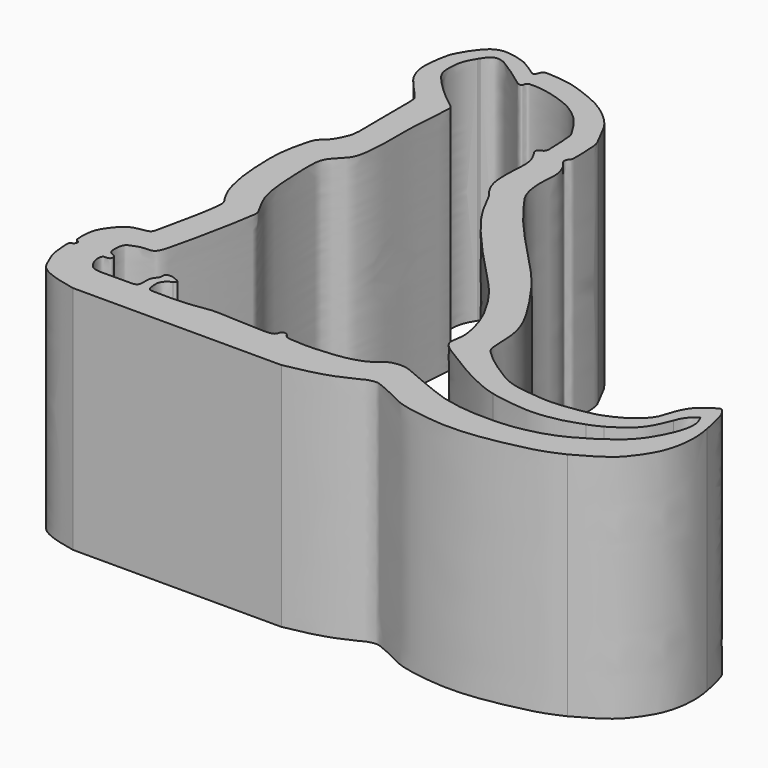
from build123d import *

# Parameters (mm, degrees)
F1_DEPTH = 10


with BuildPart() as f1:
    # F0 (on Top) → F1 (new body)
    with BuildSketch(Plane.XY):
        with BuildLine():
            add(Edge.make_bspline(
                [(-11.4531535655, 17.9316624999), (-11.3423634009, 17.8226080387), (-11.0990398713, 17.5830965577), (-10.5216537315, 17.1752428127), (-9.9832375082, 16.8116000023), (-9.3302766014, 16.5049497915), (-8.5351497911, 16.4210907342), (-7.6826916981, 16.3193589), (-6.9889404844, 16.398664447), (-6.4101964363, 16.4684482113), (-5.6925140638, 16.6154358699), (-5.2172506174, 16.8300922836), (-4.737926802, 17.0715715686), (-4.3068785624, 17.4497022766), (-4.1346039941, 17.6858196333), (-4.0643941611, 17.826827243)],
                knots=[0, 0, 0, 0, 0.042419574, 0.0931642308, 0.1423699622, 0.1931044872, 0.2473970709, 0.3037382441, 0.353898392, 0.4004323317, 0.4518808925, 0.4957535606, 0.5399514919, 0.5853730988, 0.6259275813, 0.6259275813, 0.6259275813, 0.6259275813], degree=3))
            add(Edge.make_bspline(
                [(-11.4531535655, 17.9316624999), (-11.5353278284, 18.0013325693), (-11.599494506, 18.1546413097), (-11.6392459174, 18.4329153399), (-11.6321864133, 19.5729774369), (-12.121309762, 20.7408570607), (-13.2308142182, 22.3617998661), (-13.8442255961, 23.2013966392), (-16.3773954957, 25.7550440824), (-17.205806736, 26.9338284954), (-17.893694871, 27.7744469667), (-17.9002010475, 29.021400573), (-17.8184822247, 29.5057983061), (-17.9897855014, 30.0497916449), (-18.1881615527, 30.275766195), (-18.2946934326, 30.4049965252), (-18.2620452332, 30.5813836452), (-18.1277397895, 30.6574477694), (-18.1285761686, 31.0906791932), (-18.1624494507, 31.9344986736), (-18.2120670314, 32.1457449013), (-18.2822644711, 32.2766117752)],
                knots=[0.1821779851, 0.1821779851, 0.1821779851, 0.1821779851, 0.1987968455, 0.2156710174, 0.2494905898, 0.2877760322, 0.3323884407, 0.3678427424, 0.4293232275, 0.4698632522, 0.5029651526, 0.5385501207, 0.5620196375, 0.58602784, 0.6039449868, 0.6168302331, 0.629630365, 0.6412448386, 0.6621791519, 0.6923850095, 0.7125211911, 0.7125211911, 0.7125211911, 0.7125211911], degree=3))
            add(Edge.make_bspline(
                [(-18.2822644711, 32.2766117752), (-18.3764124539, 32.4691395294), (-18.5746716934, 32.8745694176), (-18.9547100724, 33.5767458928), (-19.8713796985, 34.3090133343), (-20.6712786085, 34.6655738311), (-21.5630569798, 34.9977244911), (-22.289607185, 35.0857544204), (-22.739681166, 35.1104890737), (-22.8902895116, 35.0922607106), (-22.9567494288, 34.9547105739), (-22.9959628259, 34.85761112), (-23.0162381196, 34.789313499), (-23.0410310579, 34.7767824349), (-23.0424862006, 34.7761286919)],
                knots=[0, 0, 0, 0, 0.0875488863, 0.1843626926, 0.3004828811, 0.4033844393, 0.5086232519, 0.6027505646, 0.6738982423, 0.7129539346, 0.7530518454, 0.7894959828, 0.8210273533, 0.8229308962, 0.8229308962, 0.8229308962, 0.8229308962], degree=3))
            add(Edge.make_bspline(
                [(-23.0424862006, 34.7761286919), (-23.0449273652, 34.7750319649), (-23.0474912695, 34.7741032154), (-23.0501528602, 34.7733159161)],
                knots=[0.8229308962, 0.8229308962, 0.8229308962, 0.8229308962, 0.8261243023, 0.8261243023, 0.8261243023, 0.8261243023], degree=3))
            add(Edge.make_bspline(
                [(-23.0501528602, 34.7733159161), (-23.0545410802, 34.7718037439), (-23.0658169935, 34.7685198591), (-23.0800204513, 34.7682348796), (-23.0884888755, 34.7688855933)],
                knots=[0.0021581351, 0.0021581351, 0.0021581351, 0.0021581351, 0.005798454, 0.0111263901, 0.0111263901, 0.0111263901, 0.0111263901], degree=3))
            add(Edge.make_bspline(
                [(-23.0884888755, 34.7688855933), (-23.1003779199, 34.7686586533), (-23.1328950749, 34.7691224435), (-23.1675617858, 34.7535809385), (-23.1907266171, 34.8047911582), (-23.2061327949, 34.8275179634)],
                knots=[0.8400573422, 0.8400573422, 0.8400573422, 0.8400573422, 0.8525582929, 0.8747680855, 0.9015857102, 0.9015857102, 0.9015857102, 0.9015857102], degree=3))
            add(Edge.make_bspline(
                [(-23.2061327949, 34.8275179634), (-23.2333559253, 34.8463304823), (-23.2647020116, 34.8687780005), (-23.2981565972, 34.8923575129)],
                knots=[0.0280714161, 0.0280714161, 0.0280714161, 0.0280714161, 0.0354838753, 0.0354838753, 0.0354838753, 0.0354838753], degree=3))
            add(Edge.make_bspline(
                [(-23.2981565972, 34.8923575129), (-23.2988767288, 34.892762275), (-23.3248742022, 34.9074866854), (-23.3553511069, 34.9290724478), (-23.3874430501, 34.9538305609)],
                knots=[0.9407451714, 0.9407451714, 0.9407451714, 0.9407451714, 0.9414461456, 0.9659304091, 0.9659304091, 0.9659304091, 0.9659304091], degree=3))
            add(Edge.make_bspline(
                [(-23.3874430501, 34.9538305609), (-23.3931059977, 34.9575991511), (-23.5183257902, 35.0402229402), (-23.6443291251, 35.1054632176), (-23.7584039569, 35.1838432252)],
                knots=[0.0418291952, 0.0418291952, 0.0418291952, 0.0418291952, 0.0430086944, 0.0678657162, 0.0678657162, 0.0678657162, 0.0678657162], degree=3))
            add(Edge.make_bspline(
                [(-26.1538624763, 34.1210328043), (-26.1307370492, 34.1751880638), (-26.0822982029, 34.2886224609), (-25.9658399245, 34.4784520857), (-25.8367286637, 34.7222051807), (-25.6728345837, 34.9333072266), (-25.4439024159, 35.211302267), (-25.2265629641, 35.3669839468), (-24.9870615601, 35.4455267206), (-24.8071553611, 35.4561515908), (-24.6253811619, 35.4452719932), (-24.4282528156, 35.4124563816), (-24.2023609898, 35.3568568595), (-23.9138114794, 35.2698461332), (-23.8380879164, 35.2283194661), (-23.7584039569, 35.1838432252)],
                knots=[0, 0, 0, 0, 0.0671677149, 0.1421214746, 0.2249641321, 0.3079903593, 0.4027612882, 0.4853187471, 0.5636684732, 0.6308045814, 0.6978681882, 0.7682230286, 0.8464364216, 0.9304502691, 1, 1, 1, 1], degree=3))
            add(Edge.make_bspline(
                [(-25.1203924417, 30.8839287609), (-25.1562608207, 30.9362134154), (-25.2475018018, 31.0692136602), (-25.5941633097, 31.4371340123), (-26.0988037641, 31.9831774136), (-26.3235628346, 32.5710825271), (-26.3308719409, 33.0580330838), (-26.267644153, 33.6751860491), (-26.1899151296, 33.9797626196), (-26.1538624763, 34.1210328043)],
                knots=[0, 0, 0, 0, 0.0919674503, 0.2339442329, 0.409585968, 0.566381973, 0.7063931007, 0.8638178216, 1, 1, 1, 1], degree=3))
            add(Edge.make_bspline(
                [(-25.1203924417, 30.8839287609), (-25.0886757261, 30.8488100619), (-25.0858553072, 30.7298281237), (-25.0605183202, 30.5414498556), (-25.0811840994, 29.4385381855), (-25.025121507, 27.8856571604), (-25.0878508685, 27.3842583921), (-25.2783239246, 27.0108607833), (-25.3896626652, 26.7964370834), (-25.5940210314, 26.5788191515), (-25.8230618275, 26.4054110505), (-25.9629958258, 25.978131493), (-26.1101708802, 25.2629515982), (-26.1930934834, 24.6887465002), (-26.1587460044, 23.5953713197), (-26.0923778546, 22.7066225224), (-25.8549842087, 21.6428561237), (-25.4792186965, 21.0084943162), (-25.2488940087, 20.7558964092), (-25.6031770536, 19.1423379832), (-25.8752014488, 17.9034210742)],
                knots=[0.445949678, 0.445949678, 0.445949678, 0.445949678, 0.4606016519, 0.4767201663, 0.5169581501, 0.5660347046, 0.5932453766, 0.6172063162, 0.6362765888, 0.6569197902, 0.677099802, 0.7025270895, 0.7352531162, 0.7651894637, 0.8048239261, 0.8421337262, 0.8826114218, 0.9145317439, 0.9341388234, 1, 1, 1, 1], degree=3))
            add(Edge.make_bspline(
                [(-25.8752014488, 17.9034210742), (-25.890226418, 17.8385940614), (-25.9181016975, 17.7183228602), (-26.0280658323, 17.6086152498), (-26.3580697207, 17.5628266856), (-26.8372170059, 17.4724464527), (-27.3412522543, 16.8823959482), (-27.5876734804, 16.3942447708), (-27.5859384154, 15.7548281184), (-27.559666492, 15.6041924875), (-27.4454298624, 15.5597037984), (-27.4091925648, 15.5164474494), (-27.40446379, 15.4213679956), (-27.4685753547, 15.3262476594), (-27.5338586836, 15.3167507729), (-27.6002461641, 15.2885968197), (-27.6332812217, 15.1859599479), (-27.5983987717, 14.8301530597), (-27.5615282937, 14.3707910049), (-27.4634080296, 14.0958808888), (-27.3264889208, 13.8151837564), (-27.1982899269, 13.4630176243), (-26.9092353443, 13.1931500637), (-26.4150422105, 13.0016663658), (-26.1029425206, 12.9146269902), (-25.6877393944, 12.8221827022), (-25.4437103868, 12.765155333)],
                knots=[0, 0, 0, 0, 0.0344863373, 0.0639855733, 0.1086241936, 0.1641824578, 0.2327490814, 0.2937225355, 0.3559622593, 0.3853098427, 0.4111499512, 0.4294614236, 0.4532568552, 0.4793434925, 0.499421999, 0.5194489997, 0.5434180278, 0.5910075895, 0.64611278, 0.688915408, 0.7331184434, 0.7813380609, 0.8313225626, 0.8883414874, 0.9343006116, 1, 1, 1, 1], degree=3))
            Line((-25.4437103868, 12.765155333), (-16.4025947478, 12.765155333))
            add(Edge.make_bspline(
                [(-16.4025947478, 12.765155333), (-16.1325477154, 12.8121301717), (-15.6410122013, 12.9046834632), (-14.9844065574, 13.0825012477), (-14.3633058233, 13.2783819833), (-13.5688307679, 13.6611160533), (-13.4493540543, 13.7432549192), (-13.1147097273, 13.8045320217), (-12.93922772, 13.7837422569), (-12.1480315577, 13.437274029), (-11.5088259607, 13.0448039918), (-10.2445374068, 12.8357133347), (-9.1498502359, 12.7336593824), (-7.965074114, 12.8220975242), (-6.8232223523, 13.03483049), (-5.6038998247, 13.3021566911), (-4.9807119282, 13.5887327234), (-4.7370914961, 13.6951681509)],
                knots=[0, 0, 0, 0, 0.0553291926, 0.1059431332, 0.158535845, 0.2156720776, 0.2406225556, 0.27495853, 0.3021246856, 0.3581217371, 0.4143329098, 0.4838231748, 0.550330998, 0.6177137492, 0.6856038145, 0.7557468163, 0.8158364686, 0.8158364686, 0.8158364686, 0.8158364686], degree=3))
            add(Edge.make_bspline(
                [(-4.7370914961, 13.6951681509), (-4.6336168572, 13.7497695407), (-4.4022190396, 13.8718733002), (-3.915698601, 14.1583931236), (-3.3189609958, 14.5578766942), (-2.8415437902, 15.1210480371), (-2.393185713, 15.8326132355), (-2.1726225731, 16.5980120919), (-2.106400575, 17.3823937336), (-2.1753231615, 17.9085416842), (-2.2190036252, 18.1177239865)],
                knots=[0, 0, 0, 0, 0.0743850462, 0.1663454691, 0.2702248812, 0.3756822507, 0.4875855348, 0.5966665154, 0.7059543766, 0.810481295, 0.810481295, 0.810481295, 0.810481295], degree=3))
            add(Edge.make_bspline(
                [(-2.2190036252, 18.1177239865), (-2.2518107461, 18.2748347059), (-2.3191938065, 18.5027389298), (-2.4290399311, 18.6979265504), (-2.5020790265, 18.7794991688), (-2.5303655878, 18.8093540446)],
                knots=[0.810481295, 0.810481295, 0.810481295, 0.810481295, 0.8889884113, 0.9480975652, 0.9842665566, 0.9842665566, 0.9842665566, 0.9842665566], degree=3))
            add(Edge.make_bspline(
                [(-2.5303655878, 18.8093540446), (-2.5426701888, 18.8223408596), (-2.5550807251, 18.8351173916), (-2.5674912613, 18.8478939235)],
                knots=[0.9842665566, 0.9842665566, 0.9842665566, 0.9842665566, 1, 1, 1, 1], degree=3))
            add(Edge.make_bspline(
                [(-4.0643941611, 17.826827243), (-3.9865836201, 17.9830999177), (-3.86768057, 18.3397290309), (-3.6416754276, 18.6704218123), (-3.3503084939, 18.8584432296), (-3.0550237105, 18.9017134543), (-2.7920699812, 18.9152360919), (-2.6246045598, 18.893669034), (-2.5674912613, 18.8478939235)],
                knots=[0.6259275813, 0.6259275813, 0.6259275813, 0.6259275813, 0.6708723716, 0.7091205339, 0.7439142078, 0.7767324746, 0.8080795091, 0.8368777612, 0.8368777612, 0.8368777612, 0.8368777612], degree=3))
        make_face()
        with BuildLine():
            add(Edge.make_bspline(
                [(-18.6367090791, 26.806615293), (-18.8379953623, 27.065709235), (-19.2790347915, 27.6334113281), (-19.1385849927, 29.1576934988), (-19.142782507, 29.5768376419), (-19.2364724588, 29.9460879236), (-19.432292799, 30.245707849), (-19.5036923614, 30.3711508025), (-19.452039249, 30.531044358), (-19.1832908953, 30.5779669697), (-19.2042061287, 31.0575192756), (-19.2501349062, 31.946730439), (-19.3048676283, 32.1518750406), (-19.8206112027, 32.9401597753), (-20.1781911638, 33.2766280139), (-20.6657936013, 33.6375280434), (-21.1987273574, 33.8502544994), (-21.8156732253, 34.0369903903), (-22.3532940037, 34.1202740074), (-22.6789525507, 34.1114092951), (-22.781036981, 34.0935154005), (-22.8442123538, 34.0064923878), (-22.836017646, 33.8992917505), (-22.9169687736, 33.8654371785), (-23.0415440189, 33.8778928228), (-23.145046001, 33.9920059469), (-24.3172951647, 34.8056332509), (-24.4709784088, 34.846264388), (-24.6665006085, 34.9235282636), (-24.8730036275, 34.8890028633), (-25.0225147118, 34.7975179285), (-25.1513236902, 34.5965507599), (-25.1965038478, 34.5278270543)],
                knots=[0, 0, 0, 0, 0.0530449929, 0.1162271616, 0.1503362798, 0.1818999441, 0.2130503431, 0.2322815435, 0.2514640261, 0.275217638, 0.3099088569, 0.3591170068, 0.3848334384, 0.4340298475, 0.4724784579, 0.512097197, 0.5519606878, 0.5941304956, 0.6332780537, 0.6623280229, 0.6782450968, 0.6944721334, 0.7106995421, 0.7248499144, 0.7417640264, 0.7633659926, 0.8252786224, 0.8481238707, 0.8706340609, 0.8940154935, 0.9161281592, 0.9453600325, 0.9453600325, 0.9453600325, 0.9453600325], degree=3))
            add(Edge.make_bspline(
                [(-18.6367090791, 26.806615293), (-18.4004431072, 26.3177446993), (-17.8214250743, 25.1196658343), (-14.9958562057, 22.1558553104), (-14.2006384351, 21.3463203299), (-13.4069219143, 20.1028170279), (-13.057819762, 19.1966099457), (-12.8449499507, 18.2061038352), (-13.1501738463, 17.4728388827), (-12.0668415899, 16.9062569537), (-11.2465699819, 16.3394149694), (-10.3042035411, 15.8914402394), (-9.8099199153, 15.6800453052), (-9.4957305118, 15.6079921871)],
                knots=[0, 0, 0, 0, 0.070520737, 0.1729047088, 0.2297494243, 0.2895443737, 0.3410861891, 0.3916345783, 0.432452015, 0.4846611235, 0.5378002653, 0.5889842833, 0.636687273, 0.636687273, 0.636687273, 0.636687273], degree=3))
            add(Edge.make_bspline(
                [(-9.4957305118, 15.6079921871), (-9.1133312834, 15.5202964964), (-8.2008881683, 15.4402897436), (-7.3081707518, 15.4279642007), (-6.2775050816, 15.7326586203), (-5.5702812914, 15.970748713), (-5.1639379173, 16.0504758378), (-5.0442288589, 16.0616629529)],
                knots=[0.636687273, 0.636687273, 0.636687273, 0.636687273, 0.6947464763, 0.7437941737, 0.7961098113, 0.8448976449, 0.8661305735, 0.8661305735, 0.8661305735, 0.8661305735], degree=3))
            add(Edge.make_bspline(
                [(-5.0442288589, 16.0616629529), (-4.9399228548, 16.1184542498), (-4.6922932366, 16.2700279948), (-4.3072979632, 16.5467521861), (-3.9111782293, 16.9402090766), (-3.6467479793, 17.4860351741), (-3.5418440062, 17.7515041171), (-3.4855501726, 17.880808562)],
                knots=[0.1116059668, 0.1116059668, 0.1116059668, 0.1116059668, 0.174466562, 0.2640043057, 0.3569942582, 0.452966765, 0.5340334981, 0.5340334981, 0.5340334981, 0.5340334981], degree=3))
            add(Edge.make_bspline(
                [(-3.4855501726, 17.880808562), (-3.4648551188, 17.9392815903), (-3.4254729985, 18.0505541605), (-3.3592609609, 18.1784369474), (-3.2239072693, 18.3745123065), (-3.075018802, 18.5162428051), (-2.960889175, 18.580902775), (-2.9049660079, 18.6125859618)],
                knots=[0, 0, 0, 0, 0.1933263651, 0.3678947746, 0.5897403457, 0.798974028, 1, 1, 1, 1], degree=3))
            add(Edge.make_bspline(
                [(-2.7946273377, 18.3692199386), (-2.7964008531, 18.3746177266), (-2.8185376651, 18.4405657555), (-2.8607845108, 18.5367806837), (-2.8920297064, 18.5903902465), (-2.9049660079, 18.6125859618)],
                knots=[0.7742104558, 0.7742104558, 0.7742104558, 0.7742104558, 0.7853442377, 0.9111270835, 1, 1, 1, 1], degree=3))
            add(Edge.make_bspline(
                [(-2.7946273377, 18.3692199386), (-2.7819962135, 18.3572528177), (-2.7467831192, 18.3156041133), (-2.6954959966, 18.2431388933), (-2.7118146433, 18.0844860008), (-2.7163067479, 18.0028985872), (-2.7269718703, 17.9558321834)],
                knots=[0.7904142153, 0.7904142153, 0.7904142153, 0.7904142153, 0.8091254065, 0.8492766078, 0.8974005007, 0.94294828, 0.94294828, 0.94294828, 0.94294828], degree=3))
            add(Edge.make_bspline(
                [(-2.7589141579, 17.8106968769), (-2.7480705925, 17.8589856053), (-2.7375212314, 17.9074088943), (-2.7269718703, 17.9558321834)],
                knots=[0.9678475586, 0.9678475586, 0.9678475586, 0.9678475586, 1, 1, 1, 1], degree=3))
            add(Edge.make_bspline(
                [(-2.8583404767, 17.4271704529), (-2.8514740504, 17.4479914895), (-2.8244370396, 17.5313499213), (-2.7886322661, 17.653954814), (-2.7657065006, 17.7682841548), (-2.7589141579, 17.8106968769)],
                knots=[0.0876086045, 0.0876086045, 0.0876086045, 0.0876086045, 0.1340096964, 0.2726867204, 0.3537768689, 0.3537768689, 0.3537768689, 0.3537768689], degree=3))
            add(Edge.make_bspline(
                [(-2.8978604823, 17.3097904772), (-2.8837879349, 17.3485058616), (-2.8706743906, 17.3876598669), (-2.8583404767, 17.4271704529)],
                knots=[0.8542372602, 0.8542372602, 0.8542372602, 0.8542372602, 0.8815008623, 0.8815008623, 0.8815008623, 0.8815008623], degree=3))
            add(Edge.make_bspline(
                [(-4.1314834672, 15.5965547193), (-4.0315274216, 15.6733263507), (-3.7778639874, 15.8777413762), (-3.4320979017, 16.2764907518), (-3.160297974, 16.7462504522), (-2.970488838, 17.1099805481), (-2.8978604823, 17.3097904772)],
                knots=[0.3513635715, 0.3513635715, 0.3513635715, 0.3513635715, 0.4468641765, 0.5821895305, 0.71352993, 0.8542372602, 0.8542372602, 0.8542372602, 0.8542372602], degree=3))
            add(Edge.make_bspline(
                [(-5.1270611584, 14.938313514), (-5.0515530743, 14.9774552199), (-4.8843674391, 15.0641205227), (-4.5469469405, 15.2867318902), (-4.3174529957, 15.4558821713), (-4.1670458139, 15.5692409199), (-4.1314834672, 15.5965547193)],
                knots=[0, 0, 0, 0, 0.092613947, 0.2050604481, 0.3173863808, 0.3513635715, 0.3513635715, 0.3513635715, 0.3513635715], degree=3))
            add(Edge.make_bspline(
                [(-5.1270611584, 14.938313514), (-5.2771142269, 14.8341591333), (-5.6563184579, 14.6364611177), (-6.2827280989, 14.3709318177), (-7.113865798, 14.1755257038), (-7.8061594564, 14.0723005413), (-8.7575945258, 14.062762844), (-9.4755779778, 14.0903441294), (-10.5171680112, 14.2640694268), (-11.0849865282, 14.495208914), (-11.6394734923, 14.7117769501), (-12.3199132485, 14.9929642703), (-12.7929010289, 15.2160549407), (-13.1693051019, 15.3094794414), (-13.6631097568, 15.2406991201), (-13.8878987376, 15.0699376691), (-14.1270175817, 14.8596805039), (-14.4365379063, 14.6998032363), (-14.946365692, 14.5441603648), (-15.4653725357, 14.4701314227), (-16.0228531057, 14.4259051639), (-16.599280406, 14.3831817298), (-17.1563207893, 14.4291134823), (-17.5765573618, 14.4432909445), (-17.6426388891, 14.6781332324), (-17.9252680634, 14.7019285451), (-17.9369295949, 14.4385445784), (-18.1966937306, 14.3022551156), (-19.2514603507, 14.3796871572), (-20.1516024839, 14.4031902832), (-20.7000563565, 14.4503697732), (-21.2012371276, 14.346136563), (-21.6956016992, 14.2977665359), (-22.2745615473, 14.2463720239), (-22.9643071169, 14.2929417537), (-23.4041762898, 14.2443440285), (-23.4357489045, 14.6405144544), (-23.4448194595, 14.9162666216), (-23.2529802358, 15.1376544408), (-23.1260398226, 15.2011345711), (-23.0670906603, 15.2306137607)],
                knots=[0.2264805435, 0.2264805435, 0.2264805435, 0.2264805435, 0.2486079389, 0.2725642119, 0.2988704638, 0.3232808251, 0.3508193168, 0.3758397165, 0.4050386993, 0.427596275, 0.4496366082, 0.4744321143, 0.4951166283, 0.5129757033, 0.5327762454, 0.5479843164, 0.5638359997, 0.5807872712, 0.6016612368, 0.6226275802, 0.6440520809, 0.6659820881, 0.6879120602, 0.7054182805, 0.7182618618, 0.7311197199, 0.7440164781, 0.7580595368, 0.787518082, 0.8155871711, 0.8365634894, 0.8567932415, 0.8769411061, 0.899021601, 0.9233900622, 0.9405536451, 0.956742594, 0.9720531433, 0.9869513902, 1, 1, 1, 1], degree=3))
            add(Edge.make_bspline(
                [(-25.2310526286, 34.4719983222), (-25.3038391294, 34.3540012216), (-25.4531529498, 34.1042935473), (-25.5721470358, 33.7092541942), (-25.587188472, 33.1298241951), (-25.4997983265, 32.7713027421), (-25.0413920552, 32.246510563), (-24.405800543, 31.6505354237), (-23.897365776, 31.2578208694), (-23.7384603201, 31.1382864161), (-23.6760367082, 30.9234858301), (-23.8646136174, 29.371515056), (-23.8160584786, 27.8408048298), (-23.8551271681, 27.1541425133), (-23.9417054048, 26.339591915), (-24.1841815052, 26.0016383593), (-24.5166982086, 25.6736562258), (-24.7714149026, 25.3473157244), (-24.8024256704, 24.6413497116), (-24.7578308739, 23.6496523325), (-24.6946622518, 22.7425708957), (-24.5195394508, 21.8598876019), (-24.0198688435, 21.0761443867), (-23.9591596225, 20.7748494681), (-24.7186554159, 17.060654472), (-24.8645659656, 16.776896027), (-25.0058611967, 16.5379639168), (-25.4743029949, 16.5886627468), (-25.828810169, 16.422282137), (-26.117255434, 16.3440434258), (-26.1701546323, 15.6477142433), (-25.960334184, 15.551537143), (-25.7824829921, 15.4608173801), (-25.7700435102, 15.2730663669), (-25.9120797072, 15.1993096117), (-26.120103391, 15.2497938765), (-26.1587468696, 14.9656310604), (-26.1025293294, 14.7432897715), (-25.9857633015, 14.511549356), (-25.8184734838, 14.331032355), (-25.6147179493, 14.2801439987), (-25.3514809746, 14.2616198502), (-24.4496681404, 14.2701286396), (-24.0407142438, 14.2676187035), (-23.8240741539, 14.3523693205), (-23.8551603339, 14.7361797958), (-23.8173415435, 15.0196417279), (-23.5949082397, 15.2256291566), (-23.6362962994, 15.4703033213), (-23.5144593574, 15.5291150345), (-23.3262235385, 15.5282810576), (-23.1721817841, 15.4584836678), (-22.9132569839, 15.3623304285), (-23.0186889838, 15.2720566209), (-23.0670906603, 15.2306137607)],
                knots=[0.0027278011, 0.0027278011, 0.0027278011, 0.0027278011, 0.0200249886, 0.0393548678, 0.0612294478, 0.0786838853, 0.1025489241, 0.1307470779, 0.1538969322, 0.1658959497, 0.1780571677, 0.2142283318, 0.2513672974, 0.2758186495, 0.3014641695, 0.3202193243, 0.3398196416, 0.3581136586, 0.3821190631, 0.4115331974, 0.439462177, 0.467632387, 0.4942257926, 0.5124318159, 0.5686189168, 0.5863858262, 0.5995567566, 0.6189060586, 0.6372612295, 0.6522652849, 0.6748270314, 0.6879979824, 0.7005384814, 0.7118123465, 0.7226500232, 0.7346799252, 0.7485649543, 0.7629617211, 0.7777715626, 0.7920285271, 0.8046940387, 0.8198234075, 0.84771286, 0.866790111, 0.878951312, 0.8961848444, 0.9120081261, 0.9274768414, 0.9408689641, 0.9504318938, 0.9627680851, 0.9755932763, 0.9887953719, 1, 1, 1, 1], degree=3))
            add(Edge.make_bspline(
                [(-25.1965038478, 34.5278270543), (-25.2109680444, 34.5058255111), (-25.2225466217, 34.4885071169), (-25.2310526286, 34.4719983222)],
                knots=[0.9453600325, 0.9453600325, 0.9453600325, 0.9453600325, 0.9547184674, 0.9547184674, 0.9547184674, 0.9547184674], degree=3))
        make_face(mode=Mode.SUBTRACT)
        with BuildLine():
            add(Edge.make_bspline(
                [(-4.0643941611, 17.826827243), (-4.0329021527, 17.9274360865), (-3.9633756818, 18.1495552272), (-3.8023122301, 18.6095361712), (-3.555300918, 19.0266262674), (-3.1821771361, 19.322271683), (-2.9551182407, 19.4661996221), (-2.846354153, 19.5351429284)],
                knots=[0, 0, 0, 0, 0.1756674888, 0.38782984, 0.6003192445, 0.8085478544, 1, 1, 1, 1], degree=3))
            add(Edge.make_bspline(
                [(-4.0643941611, 17.826827243), (-3.9865836201, 17.9830999177), (-3.86768057, 18.3397290309), (-3.6416754276, 18.6704218123), (-3.3503084939, 18.8584432296), (-3.0550237105, 18.9017134543), (-2.7920699812, 18.9152360919), (-2.6246045598, 18.893669034), (-2.5674912613, 18.8478939235)],
                knots=[0.6259275813, 0.6259275813, 0.6259275813, 0.6259275813, 0.6708723716, 0.7091205339, 0.7439142078, 0.7767324746, 0.8080795091, 0.8368777612, 0.8368777612, 0.8368777612, 0.8368777612], degree=3))
            add(Edge.make_bspline(
                [(-2.5674912613, 18.8478939235), (-2.5538474608, 18.8369587037), (-2.5415202907, 18.824000489), (-2.5303655878, 18.8093540446)],
                knots=[0.8368777612, 0.8368777612, 0.8368777612, 0.8368777612, 0.843757378, 0.843757378, 0.843757378, 0.843757378], degree=3))
            add(Edge.make_bspline(
                [(-2.2190036252, 18.1177239865), (-2.2518107461, 18.2748347059), (-2.3191938065, 18.5027389298), (-2.4290399311, 18.6979265504), (-2.5020790265, 18.7794991688), (-2.5303655878, 18.8093540446)],
                knots=[0.810481295, 0.810481295, 0.810481295, 0.810481295, 0.8889884113, 0.9480975652, 0.9842665566, 0.9842665566, 0.9842665566, 0.9842665566], degree=3))
            add(Edge.make_bspline(
                [(-2.2190036252, 18.1177239865), (-2.2295599779, 18.1909128286), (-2.2525944027, 18.350614094), (-2.3311223768, 18.6665866168), (-2.411011017, 18.9856929483), (-2.5034334632, 19.2962170954), (-2.6620392862, 19.4790050752), (-2.699362075, 19.5283454236), (-2.7892871387, 19.5677127173), (-2.8284091094, 19.5453846817), (-2.846354153, 19.5351429284)],
                knots=[0, 0, 0, 0, 0.1385698593, 0.3023655142, 0.469346878, 0.6353465435, 0.772083198, 0.8437606813, 0.9283338407, 1, 1, 1, 1], degree=3))
        make_face()
        with BuildLine():
            add(Edge.make_bspline(
                [(-9.4957305118, 15.6079921871), (-9.1133312834, 15.5202964964), (-8.2008881683, 15.4402897436), (-7.3081707518, 15.4279642007), (-6.2775050816, 15.7326586203), (-5.5702812914, 15.970748713), (-5.1639379173, 16.0504758378), (-5.0442288589, 16.0616629529)],
                knots=[0.636687273, 0.636687273, 0.636687273, 0.636687273, 0.6947464763, 0.7437941737, 0.7961098113, 0.8448976449, 0.8661305735, 0.8661305735, 0.8661305735, 0.8661305735], degree=3))
            add(Edge.make_bspline(
                [(-9.4957305118, 15.6079921871), (-9.2948678262, 15.5463206649), (-8.7000059095, 15.4649529633), (-7.7290203732, 15.3419949223), (-6.8886297907, 15.4400960431), (-6.2129135882, 15.5896585333), (-5.8190504445, 15.747745542), (-5.6177424267, 15.8075205982)],
                knots=[0, 0, 0, 0, 0.0254322528, 0.0542807701, 0.0806860867, 0.1044391847, 0.1272162238, 0.1272162238, 0.1272162238, 0.1272162238], degree=3))
            add(Edge.make_bspline(
                [(-5.6177424267, 15.8075205982), (-5.466753069, 15.8664520418), (-5.2723213776, 15.9423391137), (-5.0856063663, 16.039134218), (-5.0442288589, 16.0616629529)],
                knots=[0, 0, 0, 0, 0.0866695811, 0.1116059668, 0.1116059668, 0.1116059668, 0.1116059668], degree=3))
        make_face()
        with BuildLine():
            add(Edge.make_bspline(
                [(-2.7946273377, 18.3692199386), (-2.7819962135, 18.3572528177), (-2.7467831192, 18.3156041133), (-2.6954959966, 18.2431388933), (-2.7118146433, 18.0844860008), (-2.7163067479, 18.0028985872), (-2.7269718703, 17.9558321834)],
                knots=[0.7904142153, 0.7904142153, 0.7904142153, 0.7904142153, 0.8091254065, 0.8492766078, 0.8974005007, 0.94294828, 0.94294828, 0.94294828, 0.94294828], degree=3))
            add(Edge.make_bspline(
                [(-2.7498320277, 17.8763530796), (-2.7482850512, 17.8897743927), (-2.7401795828, 17.9706760352), (-2.7408634662, 18.0956768484), (-2.745224744, 18.1928070831), (-2.7747005451, 18.308571691), (-2.7946273377, 18.3692199386)],
                knots=[0.3956408743, 0.3956408743, 0.3956408743, 0.3956408743, 0.4214109088, 0.5516550538, 0.64911396, 0.7742104558, 0.7742104558, 0.7742104558, 0.7742104558], degree=3))
            add(Edge.make_bspline(
                [(-2.7269718703, 17.9558321834), (-2.7325770316, 17.931095966), (-2.7405247135, 17.9043172658), (-2.7498320277, 17.8763530796)],
                knots=[0.94294828, 0.94294828, 0.94294828, 0.94294828, 0.9668863692, 0.9668863692, 0.9668863692, 0.9668863692], degree=3))
        make_face()
        with BuildLine():
            add(Edge.make_bspline(
                [(-23.0884888755, 34.7688855933), (-23.1003779199, 34.7686586533), (-23.1328950749, 34.7691224435), (-23.1675617858, 34.7535809385), (-23.1907266171, 34.8047911582), (-23.2061327949, 34.8275179634)],
                knots=[0.8400573422, 0.8400573422, 0.8400573422, 0.8400573422, 0.8525582929, 0.8747680855, 0.9015857102, 0.9015857102, 0.9015857102, 0.9015857102], degree=3))
            add(Edge.make_bspline(
                [(-23.0884888755, 34.7688855933), (-23.0908912433, 34.7690701912), (-23.1071818944, 34.7707677433), (-23.1325886424, 34.7781756239), (-23.1815038199, 34.8104981332), (-23.2061327949, 34.8275179634)],
                knots=[0.0111263901, 0.0111263901, 0.0111263901, 0.0111263901, 0.0126378475, 0.0213653073, 0.0280714161, 0.0280714161, 0.0280714161, 0.0280714161], degree=3))
        make_face()
        with BuildLine():
            add(Edge.make_bspline(
                [(-2.7589141579, 17.8106968769), (-2.7480705925, 17.8589856053), (-2.7375212314, 17.9074088943), (-2.7269718703, 17.9558321834)],
                knots=[0.9678475586, 0.9678475586, 0.9678475586, 0.9678475586, 1, 1, 1, 1], degree=3))
            add(Edge.make_bspline(
                [(-2.7269718703, 17.9558321834), (-2.7325770316, 17.931095966), (-2.7405247135, 17.9043172658), (-2.7498320277, 17.8763530796)],
                knots=[0.94294828, 0.94294828, 0.94294828, 0.94294828, 0.9668863692, 0.9668863692, 0.9668863692, 0.9668863692], degree=3))
            add(Edge.make_bspline(
                [(-2.7589141579, 17.8106968769), (-2.7554075091, 17.8325930808), (-2.7523451261, 17.854549852), (-2.7498320277, 17.8763530796)],
                knots=[0.3537768689, 0.3537768689, 0.3537768689, 0.3537768689, 0.3956408743, 0.3956408743, 0.3956408743, 0.3956408743], degree=3))
        make_face()
        with BuildLine():
            add(Edge.make_bspline(
                [(-23.2981565972, 34.8923575129), (-23.2988767288, 34.892762275), (-23.3248742022, 34.9074866854), (-23.3553511069, 34.9290724478), (-23.3874430501, 34.9538305609)],
                knots=[0.9407451714, 0.9407451714, 0.9407451714, 0.9407451714, 0.9414461456, 0.9659304091, 0.9659304091, 0.9659304091, 0.9659304091], degree=3))
            add(Edge.make_bspline(
                [(-23.2981565972, 34.8923575129), (-23.3267948721, 34.9125423858), (-23.3569782443, 34.9335567781), (-23.3874430501, 34.9538305609)],
                knots=[0.0354838753, 0.0354838753, 0.0354838753, 0.0354838753, 0.0418291952, 0.0418291952, 0.0418291952, 0.0418291952], degree=3))
        make_face()
        with BuildLine():
            add(Edge.make_bspline(
                [(-2.5674912613, 18.8478939235), (-2.5538474608, 18.8369587037), (-2.5415202907, 18.824000489), (-2.5303655878, 18.8093540446)],
                knots=[0.8368777612, 0.8368777612, 0.8368777612, 0.8368777612, 0.843757378, 0.843757378, 0.843757378, 0.843757378], degree=3))
            add(Edge.make_bspline(
                [(-2.5303655878, 18.8093540446), (-2.5426701888, 18.8223408596), (-2.5550807251, 18.8351173916), (-2.5674912613, 18.8478939235)],
                knots=[0.9842665566, 0.9842665566, 0.9842665566, 0.9842665566, 1, 1, 1, 1], degree=3))
        make_face()
        with BuildLine():
            add(Edge.make_bspline(
                [(-2.8978604823, 17.3097904772), (-2.8845826334, 17.3488246564), (-2.8713047844, 17.3878588357), (-2.8583404767, 17.4271704529)],
                knots=[0, 0, 0, 0, 0.0876086045, 0.0876086045, 0.0876086045, 0.0876086045], degree=3))
            add(Edge.make_bspline(
                [(-2.8978604823, 17.3097904772), (-2.8837879349, 17.3485058616), (-2.8706743906, 17.3876598669), (-2.8583404767, 17.4271704529)],
                knots=[0.8542372602, 0.8542372602, 0.8542372602, 0.8542372602, 0.8815008623, 0.8815008623, 0.8815008623, 0.8815008623], degree=3))
        make_face()
        with BuildLine():
            add(Edge.make_bspline(
                [(-25.1965038478, 34.5278270543), (-25.2080389497, 34.5092168777), (-25.2195740516, 34.4906067012), (-25.2310526286, 34.4719983222)],
                knots=[0, 0, 0, 0, 0.0027278011, 0.0027278011, 0.0027278011, 0.0027278011], degree=3))
            add(Edge.make_bspline(
                [(-25.1965038478, 34.5278270543), (-25.2109680444, 34.5058255111), (-25.2225466217, 34.4885071169), (-25.2310526286, 34.4719983222)],
                knots=[0.9453600325, 0.9453600325, 0.9453600325, 0.9453600325, 0.9547184674, 0.9547184674, 0.9547184674, 0.9547184674], degree=3))
        make_face()
    extrude(amount=F1_DEPTH)


solid = f1.part
